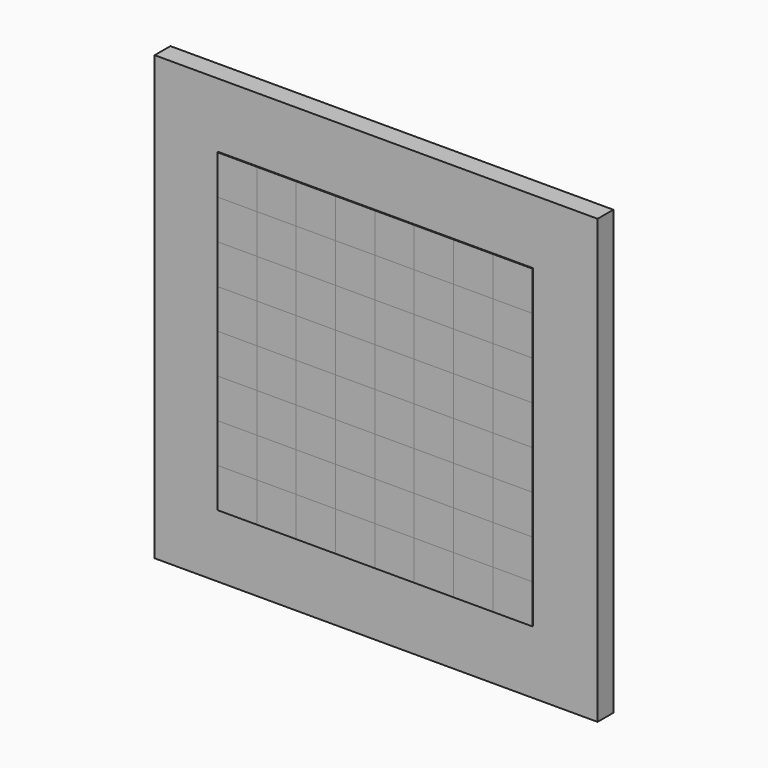
from build123d import *

# Parameters (mm, degrees)
F0_W     = 450
F0_H     = 450
F1_DEPTH = 20
F2_W     = 40
F2_H     = 40
F3_DEPTH = 1
F4_DEPTH = 1


# Not quite as in the source:
# - a feature names something its author has since deleted; it is built from what else it names


with BuildPart() as f1:
    # F0 (on Front) → F1 (new body)
    with BuildSketch(Plane.XZ):
        with Locations((-225, 225)):
            Rectangle(F0_W, F0_H)
    extrude(amount=F1_DEPTH)


with BuildPart() as f3:
    # F2 (on face) → F3 (new body)
    with BuildSketch(Plane.XZ.offset(20)):
        with Locations((-365.4713698072, 324.5286301928)):
            Rectangle(F2_W, F2_H)
    extrude(amount=F3_DEPTH)


with BuildPart() as f3b:
    # F2 (on face) → F3, piece 2 (new body)
    with BuildSketch(Plane.XZ.offset(20)):
        with Locations((-325.4713698072, 364.5286301928)):
            Rectangle(F2_W, F2_H)
    extrude(amount=F3_DEPTH)


with BuildPart() as f3c:
    # F2 (on face) → F3, piece 3 (new body)
    with BuildSketch(Plane.XZ.offset(20)):
        with Locations((-285.4713698072, 324.5286301928)):
            Rectangle(F2_W, F2_H)
    extrude(amount=F3_DEPTH)


with BuildPart() as f3d:
    # F2 (on face) → F3, piece 4 (new body)
    with BuildSketch(Plane.XZ.offset(20)):
        with Locations((-245.4713698072, 364.5286301928)):
            Rectangle(F2_W, F2_H)
    extrude(amount=F3_DEPTH)


with BuildPart() as f3e:
    # F2 (on face) → F3, piece 5 (new body)
    with BuildSketch(Plane.XZ.offset(20)):
        with Locations((-205.4713698072, 324.5286301928)):
            Rectangle(F2_W, F2_H)
    extrude(amount=F3_DEPTH)


with BuildPart() as f3f:
    # F2 (on face) → F3, piece 6 (new body)
    with BuildSketch(Plane.XZ.offset(20)):
        with Locations((-165.4713698072, 364.5286301928)):
            Rectangle(F2_W, F2_H)
    extrude(amount=F3_DEPTH)


with BuildPart() as f3g:
    # F2 (on face) → F3, piece 7 (new body)
    with BuildSketch(Plane.XZ.offset(20)):
        with Locations((-125.4713698072, 324.5286301928)):
            Rectangle(F2_W, F2_H)
    extrude(amount=F3_DEPTH)


with BuildPart() as f3h:
    # F2 (on face) → F3, piece 8 (new body)
    with BuildSketch(Plane.XZ.offset(20)):
        with Locations((-85.4713698072, 364.5286301928)):
            Rectangle(F2_W, F2_H)
    extrude(amount=F3_DEPTH)


with BuildPart() as f3i:
    # F2 (on face) → F3, piece 9 (new body)
    with BuildSketch(Plane.XZ.offset(20)):
        with Locations((-85.4713698072, 284.5286301928)):
            Rectangle(F2_W, F2_H)
    extrude(amount=F3_DEPTH)


with BuildPart() as f3j:
    # F2 (on face) → F3, piece 10 (new body)
    with BuildSketch(Plane.XZ.offset(20)):
        with Locations((-165.4713698072, 284.5286301928)):
            Rectangle(F2_W, F2_H)
    extrude(amount=F3_DEPTH)


with BuildPart() as f3k:
    # F2 (on face) → F3, piece 11 (new body)
    with BuildSketch(Plane.XZ.offset(20)):
        with Locations((-245.4713698072, 284.5286301928)):
            Rectangle(F2_W, F2_H)
    extrude(amount=F3_DEPTH)


with BuildPart() as f3l:
    # F2 (on face) → F3, piece 12 (new body)
    with BuildSketch(Plane.XZ.offset(20)):
        with Locations((-325.4713698072, 284.5286301928)):
            Rectangle(F2_W, F2_H)
    extrude(amount=F3_DEPTH)


with BuildPart() as f3m:
    # F2 (on face) → F3, piece 13 (new body)
    with BuildSketch(Plane.XZ.offset(20)):
        with Locations((-365.4713698072, 244.5286301928)):
            Rectangle(F2_W, F2_H)
    extrude(amount=F3_DEPTH)


with BuildPart() as f3n:
    # F2 (on face) → F3, piece 14 (new body)
    with BuildSketch(Plane.XZ.offset(20)):
        with Locations((-285.4713698072, 244.5286301928)):
            Rectangle(F2_W, F2_H)
    extrude(amount=F3_DEPTH)


with BuildPart() as f3o:
    # F2 (on face) → F3, piece 15 (new body)
    with BuildSketch(Plane.XZ.offset(20)):
        with Locations((-205.4713698072, 244.5286301928)):
            Rectangle(F2_W, F2_H)
    extrude(amount=F3_DEPTH)


with BuildPart() as f3p:
    # F2 (on face) → F3, piece 16 (new body)
    with BuildSketch(Plane.XZ.offset(20)):
        with Locations((-125.4713698072, 244.5286301928)):
            Rectangle(F2_W, F2_H)
    extrude(amount=F3_DEPTH)


with BuildPart() as f3q:
    # F2 (on face) → F3, piece 17 (new body)
    with BuildSketch(Plane.XZ.offset(20)):
        with Locations((-85.4713698072, 204.5286301928)):
            Rectangle(F2_W, F2_H)
    extrude(amount=F3_DEPTH)


with BuildPart() as f3r:
    # F2 (on face) → F3, piece 18 (new body)
    with BuildSketch(Plane.XZ.offset(20)):
        with Locations((-165.4713698072, 204.5286301928)):
            Rectangle(F2_W, F2_H)
    extrude(amount=F3_DEPTH)


with BuildPart() as f3s:
    # F2 (on face) → F3, piece 19 (new body)
    with BuildSketch(Plane.XZ.offset(20)):
        with Locations((-245.4713698072, 204.5286301928)):
            Rectangle(F2_W, F2_H)
    extrude(amount=F3_DEPTH)


with BuildPart() as f3t:
    # F2 (on face) → F3, piece 20 (new body)
    with BuildSketch(Plane.XZ.offset(20)):
        with Locations((-325.4713698072, 204.5286301928)):
            Rectangle(F2_W, F2_H)
    extrude(amount=F3_DEPTH)


with BuildPart() as f3u:
    # F2 (on face) → F3, piece 21 (new body)
    with BuildSketch(Plane.XZ.offset(20)):
        with Locations((-365.4713698072, 164.5286301928)):
            Rectangle(F2_W, F2_H)
    extrude(amount=F3_DEPTH)


with BuildPart() as f3v:
    # F2 (on face) → F3, piece 22 (new body)
    with BuildSketch(Plane.XZ.offset(20)):
        with Locations((-285.4713698072, 164.5286301928)):
            Rectangle(F2_W, F2_H)
    extrude(amount=F3_DEPTH)


with BuildPart() as f3w:
    # F2 (on face) → F3, piece 23 (new body)
    with BuildSketch(Plane.XZ.offset(20)):
        with Locations((-205.4713698072, 164.5286301928)):
            Rectangle(F2_W, F2_H)
    extrude(amount=F3_DEPTH)


with BuildPart() as f3x:
    # F2 (on face) → F3, piece 24 (new body)
    with BuildSketch(Plane.XZ.offset(20)):
        with Locations((-125.4713698072, 164.5286301928)):
            Rectangle(F2_W, F2_H)
    extrude(amount=F3_DEPTH)


with BuildPart() as f3y:
    # F2 (on face) → F3, piece 25 (new body)
    with BuildSketch(Plane.XZ.offset(20)):
        with Locations((-85.4713698072, 124.5286301928)):
            Rectangle(F2_W, F2_H)
    extrude(amount=F3_DEPTH)


with BuildPart() as f3z:
    # F2 (on face) → F3, piece 26 (new body)
    with BuildSketch(Plane.XZ.offset(20)):
        with Locations((-165.4713698072, 124.5286301928)):
            Rectangle(F2_W, F2_H)
    extrude(amount=F3_DEPTH)


with BuildPart() as f3ba:
    # F2 (on face) → F3, piece 27 (new body)
    with BuildSketch(Plane.XZ.offset(20)):
        with Locations((-245.4713698072, 124.5286301928)):
            Rectangle(F2_W, F2_H)
    extrude(amount=F3_DEPTH)


with BuildPart() as f3bb:
    # F2 (on face) → F3, piece 28 (new body)
    with BuildSketch(Plane.XZ.offset(20)):
        with Locations((-325.4713698072, 124.5286301928)):
            Rectangle(F2_W, F2_H)
    extrude(amount=F3_DEPTH)


with BuildPart() as f3bc:
    # F2 (on face) → F3, piece 29 (new body)
    with BuildSketch(Plane.XZ.offset(20)):
        with Locations((-365.4713698072, 84.5286301928)):
            Rectangle(F2_W, F2_H)
    extrude(amount=F3_DEPTH)


with BuildPart() as f3bd:
    # F2 (on face) → F3, piece 30 (new body)
    with BuildSketch(Plane.XZ.offset(20)):
        with Locations((-285.4713698072, 84.5286301928)):
            Rectangle(F2_W, F2_H)
    extrude(amount=F3_DEPTH)


with BuildPart() as f3be:
    # F2 (on face) → F3, piece 31 (new body)
    with BuildSketch(Plane.XZ.offset(20)):
        with Locations((-205.4713698072, 84.5286301928)):
            Rectangle(F2_W, F2_H)
    extrude(amount=F3_DEPTH)


with BuildPart() as f3bf:
    # F2 (on face) → F3, piece 32 (new body)
    with BuildSketch(Plane.XZ.offset(20)):
        with Locations((-125.4713698072, 84.5286301928)):
            Rectangle(F2_W, F2_H)
    extrude(amount=F3_DEPTH)


with BuildPart() as f4:
    # F2 (on face) → F4 (new body)
    with BuildSketch(Plane.XZ.offset(20)):
        with Locations((-365.4713698072, 364.5286301928)):
            Rectangle(F2_W, F2_H)
    extrude(amount=F4_DEPTH)


with BuildPart() as f4b:
    # F2 (on face) → F4, piece 2 (new body)
    with BuildSketch(Plane.XZ.offset(20)):
        with Locations((-325.4713698072, 324.5286301928)):
            Rectangle(F2_W, F2_H)
    extrude(amount=F4_DEPTH)


with BuildPart() as f4c:
    # F2 (on face) → F4, piece 3 (new body)
    with BuildSketch(Plane.XZ.offset(20)):
        with Locations((-285.4713698072, 364.5286301928)):
            Rectangle(F2_W, F2_H)
    extrude(amount=F4_DEPTH)


with BuildPart() as f4d:
    # F2 (on face) → F4, piece 4 (new body)
    with BuildSketch(Plane.XZ.offset(20)):
        with Locations((-365.4713698072, 284.5286301928)):
            Rectangle(F2_W, F2_H)
    extrude(amount=F4_DEPTH)


with BuildPart() as f4e:
    # F2 (on face) → F4, piece 5 (new body)
    with BuildSketch(Plane.XZ.offset(20)):
        with Locations((-285.4713698072, 284.5286301928)):
            Rectangle(F2_W, F2_H)
    extrude(amount=F4_DEPTH)


with BuildPart() as f4f:
    # F2 (on face) → F4, piece 6 (new body)
    with BuildSketch(Plane.XZ.offset(20)):
        with Locations((-245.4713698072, 324.5286301928)):
            Rectangle(F2_W, F2_H)
    extrude(amount=F4_DEPTH)


with BuildPart() as f4g:
    # F2 (on face) → F4, piece 7 (new body)
    with BuildSketch(Plane.XZ.offset(20)):
        with Locations((-205.4713698072, 364.5286301928)):
            Rectangle(F2_W, F2_H)
    extrude(amount=F4_DEPTH)


with BuildPart() as f4h:
    # F2 (on face) → F4, piece 8 (new body)
    with BuildSketch(Plane.XZ.offset(20)):
        with Locations((-205.4713698072, 284.5286301928)):
            Rectangle(F2_W, F2_H)
    extrude(amount=F4_DEPTH)


with BuildPart() as f4i:
    # F2 (on face) → F4, piece 9 (new body)
    with BuildSketch(Plane.XZ.offset(20)):
        with Locations((-165.4713698072, 324.5286301928)):
            Rectangle(F2_W, F2_H)
    extrude(amount=F4_DEPTH)


with BuildPart() as f4j:
    # F2 (on face) → F4, piece 10 (new body)
    with BuildSketch(Plane.XZ.offset(20)):
        with Locations((-125.4713698072, 364.5286301928)):
            Rectangle(F2_W, F2_H)
    extrude(amount=F4_DEPTH)


with BuildPart() as f4k:
    # F2 (on face) → F4, piece 11 (new body)
    with BuildSketch(Plane.XZ.offset(20)):
        with Locations((-125.4713698072, 284.5286301928)):
            Rectangle(F2_W, F2_H)
    extrude(amount=F4_DEPTH)


with BuildPart() as f4l:
    # F2 (on face) → F4, piece 12 (new body)
    with BuildSketch(Plane.XZ.offset(20)):
        with Locations((-85.4713698072, 324.5286301928)):
            Rectangle(F2_W, F2_H)
    extrude(amount=F4_DEPTH)


with BuildPart() as f4m:
    # F2 (on face) → F4, piece 13 (new body)
    with BuildSketch(Plane.XZ.offset(20)):
        with Locations((-85.4713698072, 244.5286301928)):
            Rectangle(F2_W, F2_H)
    extrude(amount=F4_DEPTH)


with BuildPart() as f4n:
    # F2 (on face) → F4, piece 14 (new body)
    with BuildSketch(Plane.XZ.offset(20)):
        with Locations((-165.4713698072, 244.5286301928)):
            Rectangle(F2_W, F2_H)
    extrude(amount=F4_DEPTH)


with BuildPart() as f4o:
    # F2 (on face) → F4, piece 15 (new body)
    with BuildSketch(Plane.XZ.offset(20)):
        with Locations((-245.4713698072, 244.5286301928)):
            Rectangle(F2_W, F2_H)
    extrude(amount=F4_DEPTH)


with BuildPart() as f4p:
    # F2 (on face) → F4, piece 16 (new body)
    with BuildSketch(Plane.XZ.offset(20)):
        with Locations((-325.4713698072, 244.5286301928)):
            Rectangle(F2_W, F2_H)
    extrude(amount=F4_DEPTH)


with BuildPart() as f4q:
    # F2 (on face) → F4, piece 17 (new body)
    with BuildSketch(Plane.XZ.offset(20)):
        with Locations((-365.4713698072, 204.5286301928)):
            Rectangle(F2_W, F2_H)
    extrude(amount=F4_DEPTH)


with BuildPart() as f4r:
    # F2 (on face) → F4, piece 18 (new body)
    with BuildSketch(Plane.XZ.offset(20)):
        with Locations((-285.4713698072, 204.5286301928)):
            Rectangle(F2_W, F2_H)
    extrude(amount=F4_DEPTH)


with BuildPart() as f4s:
    # F2 (on face) → F4, piece 19 (new body)
    with BuildSketch(Plane.XZ.offset(20)):
        with Locations((-205.4713698072, 204.5286301928)):
            Rectangle(F2_W, F2_H)
    extrude(amount=F4_DEPTH)


with BuildPart() as f4t:
    # F2 (on face) → F4, piece 20 (new body)
    with BuildSketch(Plane.XZ.offset(20)):
        with Locations((-125.4713698072, 204.5286301928)):
            Rectangle(F2_W, F2_H)
    extrude(amount=F4_DEPTH)


with BuildPart() as f4u:
    # F2 (on face) → F4, piece 21 (new body)
    with BuildSketch(Plane.XZ.offset(20)):
        with Locations((-85.4713698072, 164.5286301928)):
            Rectangle(F2_W, F2_H)
    extrude(amount=F4_DEPTH)


with BuildPart() as f4v:
    # F2 (on face) → F4, piece 22 (new body)
    with BuildSketch(Plane.XZ.offset(20)):
        with Locations((-165.4713698072, 164.5286301928)):
            Rectangle(F2_W, F2_H)
    extrude(amount=F4_DEPTH)


with BuildPart() as f4w:
    # F2 (on face) → F4, piece 23 (new body)
    with BuildSketch(Plane.XZ.offset(20)):
        with Locations((-245.4713698072, 164.5286301928)):
            Rectangle(F2_W, F2_H)
    extrude(amount=F4_DEPTH)


with BuildPart() as f4x:
    # F2 (on face) → F4, piece 24 (new body)
    with BuildSketch(Plane.XZ.offset(20)):
        with Locations((-325.4713698072, 164.5286301928)):
            Rectangle(F2_W, F2_H)
    extrude(amount=F4_DEPTH)


with BuildPart() as f4y:
    # F2 (on face) → F4, piece 25 (new body)
    with BuildSketch(Plane.XZ.offset(20)):
        with Locations((-365.4713698072, 124.5286301928)):
            Rectangle(F2_W, F2_H)
    extrude(amount=F4_DEPTH)


with BuildPart() as f4z:
    # F2 (on face) → F4, piece 26 (new body)
    with BuildSketch(Plane.XZ.offset(20)):
        with Locations((-285.4713698072, 124.5286301928)):
            Rectangle(F2_W, F2_H)
    extrude(amount=F4_DEPTH)


with BuildPart() as f4ba:
    # F2 (on face) → F4, piece 27 (new body)
    with BuildSketch(Plane.XZ.offset(20)):
        with Locations((-205.4713698072, 124.5286301928)):
            Rectangle(F2_W, F2_H)
    extrude(amount=F4_DEPTH)


with BuildPart() as f4bb:
    # F2 (on face) → F4, piece 28 (new body)
    with BuildSketch(Plane.XZ.offset(20)):
        with Locations((-125.4713698072, 124.5286301928)):
            Rectangle(F2_W, F2_H)
    extrude(amount=F4_DEPTH)


with BuildPart() as f4bc:
    # F2 (on face) → F4, piece 29 (new body)
    with BuildSketch(Plane.XZ.offset(20)):
        with Locations((-85.4713698072, 84.5286301928)):
            Rectangle(F2_W, F2_H)
    extrude(amount=F4_DEPTH)


with BuildPart() as f4bd:
    # F2 (on face) → F4, piece 30 (new body)
    with BuildSketch(Plane.XZ.offset(20)):
        with Locations((-165.4713698072, 84.5286301928)):
            Rectangle(F2_W, F2_H)
    extrude(amount=F4_DEPTH)


with BuildPart() as f4be:
    # F2 (on face) → F4, piece 31 (new body)
    with BuildSketch(Plane.XZ.offset(20)):
        with Locations((-245.4713698072, 84.5286301928)):
            Rectangle(F2_W, F2_H)
    extrude(amount=F4_DEPTH)


with BuildPart() as f4bf:
    # F2 (on face) → F4, piece 32 (new body)
    with BuildSketch(Plane.XZ.offset(20)):
        with Locations((-325.4713698072, 84.5286301928)):
            Rectangle(F2_W, F2_H)
    extrude(amount=F4_DEPTH)


solid = Compound([f1.part, f3.part, f3b.part, f3c.part, f3d.part, f3e.part, f3f.part, f3g.part, f3h.part, f3i.part, f3j.part, f3k.part, f3l.part, f3m.part, f3n.part, f3o.part, f3p.part, f3q.part, f3r.part, f3s.part, f3t.part, f3u.part, f3v.part, f3w.part, f3x.part, f3y.part, f3z.part, f3ba.part, f3bb.part, f3bc.part, f3bd.part, f3be.part, f3bf.part, f4.part, f4b.part, f4c.part, f4d.part, f4e.part, f4f.part, f4g.part, f4h.part, f4i.part, f4j.part, f4k.part, f4l.part, f4m.part, f4n.part, f4o.part, f4p.part, f4q.part, f4r.part, f4s.part, f4t.part, f4u.part, f4v.part, f4w.part, f4x.part, f4y.part, f4z.part, f4ba.part, f4bb.part, f4bc.part, f4bd.part, f4be.part, f4bf.part])
